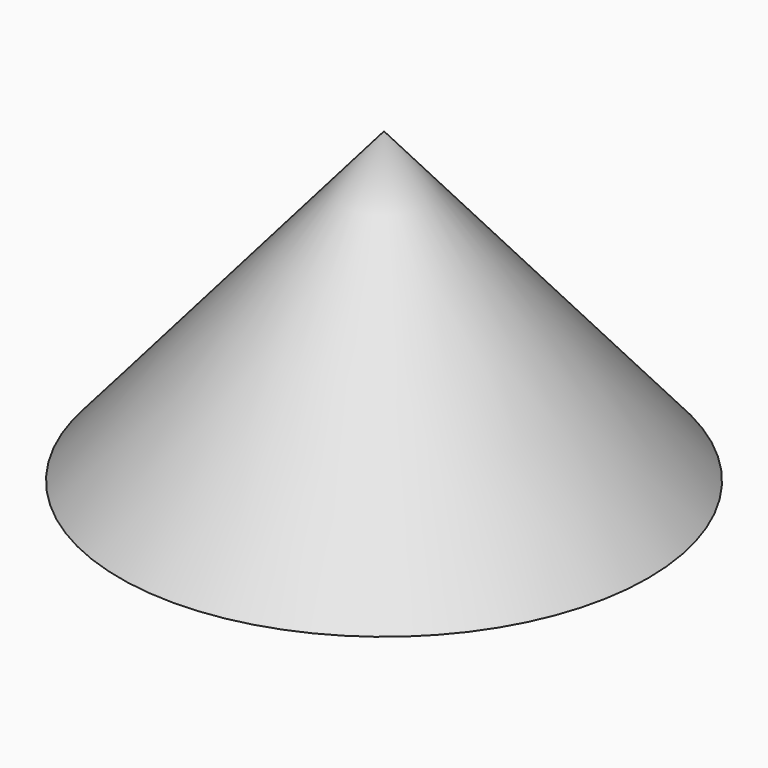
from build123d import *


# Not quite as in the source:
# - the program builds the solid bodies; features that only make, move or delete a surface that nothing else refers to are left out


with BuildPart() as f1:
    # F0 (on Front) → F1 (revolve)
    with BuildSketch(Plane.XZ):
        Polygon((0, 45.3088991344), (-38.8689748943, 0), (0, 0), align=None)
    revolve(axis=Axis((0, 0, 22.6544495672), (0, 0, 1)))


solid = f1.part
